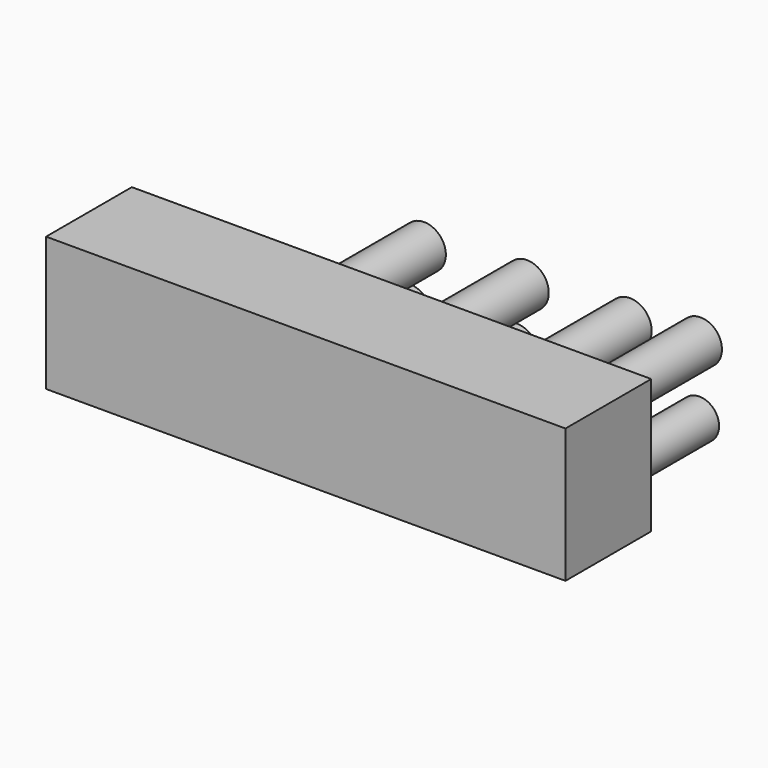
from build123d import *

# Parameters (mm, degrees)
F0_W     = 123.0572126806
F0_H     = 31.779345125
F1_DEPTH = 25.4
F2_R     = 5.0577468646
F3_DEPTH = 25.4
F4_R     = 4.6656704546
F5_DEPTH = 25.4
F6_R     = 5.7177995667
F7_DEPTH = 25.4
F8_R     = 5.1626495497
F9_DEPTH = 25.4


# Not quite as in the source:
# - a feature names something its author has since deleted; it is built from what else it names


with BuildPart() as f1:
    # F0 (on Front) → F1 (new body)
    with BuildSketch(Plane.XZ):
        with Locations((-2.7109328657, 53.5084176809)):
            Rectangle(F0_W, F0_H)
    extrude(amount=F1_DEPTH)

    # F4 (on face) → F5 (join)
    with BuildSketch(Plane(origin=(0, 0, 0), x_dir=(-1, 0, 0), z_dir=(0, 1, 0))):
        with Locations((-49.9067381024, 47.8602088988)):
            Circle(F4_R)
    extrude(amount=F5_DEPTH)


with BuildPart() as f3:
    # F2 (on face) → F3 (new body)
    with BuildSketch(Plane(origin=(0, 0, 0), x_dir=(-1, 0, 0), z_dir=(0, 1, 0))):
        with Locations((-50.196506083, 64.0703812242)):
            Circle(F2_R)
    extrude(amount=F3_DEPTH)


with BuildPart() as f7:
    # F6 (on face) → F7 (new body)
    with BuildSketch(Plane(origin=(0, 0, 0), x_dir=(-1, 0, 0), z_dir=(0, 1, 0))):
        with Locations((-31.9035984576, 47.9707233608)):
            Circle(F6_R)
    extrude(amount=F7_DEPTH)


with BuildPart() as f7b:
    # F6 (on face) → F7, piece 2 (new body)
    with BuildSketch(Plane(origin=(0, 0, 0), x_dir=(-1, 0, 0), z_dir=(0, 1, 0))):
        with Locations((-6.5035984576, 47.9707233608)):
            Circle(F6_R)
    extrude(amount=F7_DEPTH)


with BuildPart() as f7c:
    # F6 (on face) → F7, piece 3 (new body)
    with BuildSketch(Plane(origin=(0, 0, 0), x_dir=(-1, 0, 0), z_dir=(0, 1, 0))):
        with Locations((18.8964015424, 47.9707233608)):
            Circle(F6_R)
    extrude(amount=F7_DEPTH)


with BuildPart() as f9:
    # F8 (on face) → F9 (new body)
    with BuildSketch(Plane(origin=(0, 0, 0), x_dir=(-1, 0, 0), z_dir=(0, 1, 0))):
        with Locations((-33.4423966706, 62.5433772802)):
            Circle(F8_R)
    extrude(amount=F9_DEPTH)


with BuildPart() as f9b:
    # F8 (on face) → F9, piece 2 (new body)
    with BuildSketch(Plane(origin=(0, 0, 0), x_dir=(-1, 0, 0), z_dir=(0, 1, 0))):
        with Locations((-9.0583966706, 62.5433772802)):
            Circle(F8_R)
    extrude(amount=F9_DEPTH)


with BuildPart() as f9c:
    # F8 (on face) → F9, piece 3 (new body)
    with BuildSketch(Plane(origin=(0, 0, 0), x_dir=(-1, 0, 0), z_dir=(0, 1, 0))):
        with Locations((15.3256033294, 62.5433772802)):
            Circle(F8_R)
    extrude(amount=F9_DEPTH)


solid = Compound([f1.part, f3.part, f7.part, f7b.part, f7c.part, f9.part, f9b.part, f9c.part])
